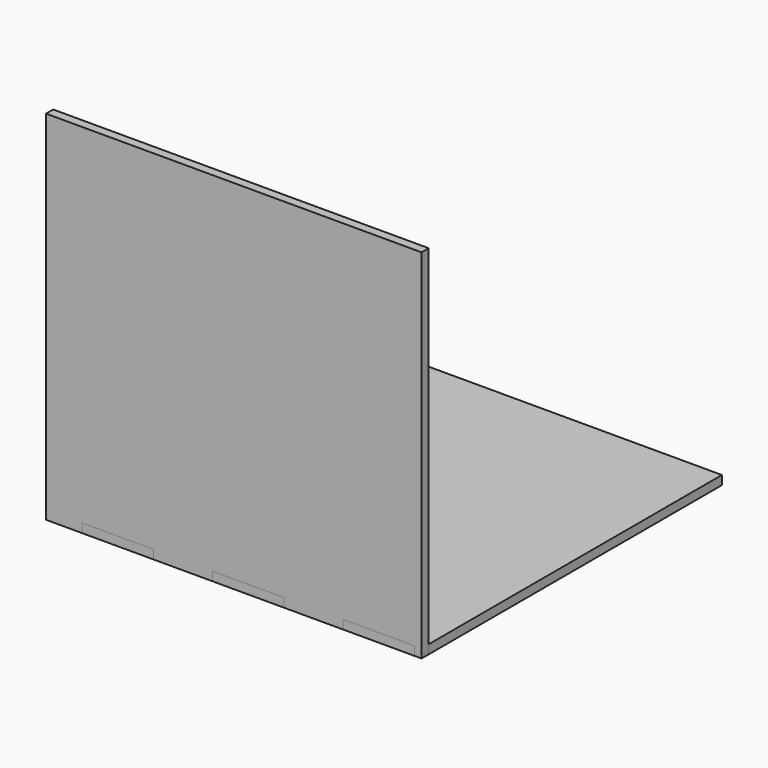
from build123d import *

# Parameters (mm, degrees)
F0_W     = 133.35
F0_H     = 133.35
F1_DEPTH = 3.175
F2_W     = 133.35
F2_H     = 3.175
F3_DEPTH = 127
F4_W     = 25.4
F4_H     = 3.175
F5_DEPTH = 25.4


with BuildPart() as f1:
    # F0 (on Top) → F1 (new body)
    with BuildSketch(Plane.XY):
        Rectangle(F0_W, F0_H)
    extrude(amount=F1_DEPTH)


with BuildPart() as f3:
    # F2 (on Top) → F3 (new body)
    with BuildSketch(Plane.XY):
        with Locations((0, -65.0875)):
            Rectangle(F2_W, F2_H)
    extrude(amount=F3_DEPTH)

    # F4 (on face) → F5 (cut)
    with BuildSketch(Plane.XZ.offset(66.675)):
        with Locations((-41.1575537503, 1.5875)):
            Rectangle(F4_W, F4_H)
        with Locations((5.1974462497, 1.5875)):
            Rectangle(F4_W, F4_H)
        with Locations((51.5524462497, 1.5875)):
            Rectangle(F4_W, F4_H)
    extrude(amount=-F5_DEPTH, mode=Mode.SUBTRACT)


with BuildPart() as f1_1:
    add(f1.part)

    # F6: cut F3
    add(f3.part, mode=Mode.SUBTRACT)


solid = Compound([f3.part, f1_1.part])
